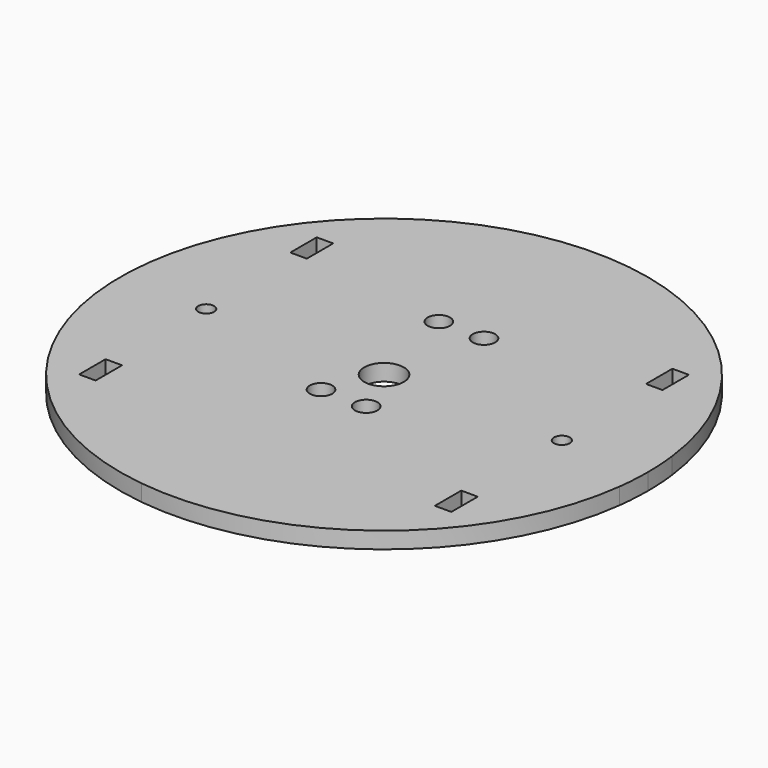
from build123d import *

# Parameters (mm, degrees)
F0_W     = 3.175
F0_H     = 6.35
F0_R     = 1.524
F0_R_2   = 2.159
F0_R_3   = 3.81
F1_DEPTH = 3.175


# Not quite as in the source:
# - a length typed as a fraction of an inch, garbled in the dataset ("3 / 203.2 mm" for 3/8 in), is restored


with BuildPart() as f1:
    # F0 (on Top) → F1 (new body)
    with BuildSketch(Plane.XY):
        with BuildLine():
            ThreePointArc((-50.403125, 6.3375855209), (-50.8, 0), (-50.403125, -6.3375855209))
            ThreePointArc((-50.403125, -6.3375855209), (-35.9210244843, -35.9210244843), (-6.3375855209, -50.403125))
            ThreePointArc((-6.3375855209, -50.403125), (0, -50.8), (6.3375855209, -50.403125))
            ThreePointArc((6.3375855209, -50.403125), (35.9210244843, -35.9210244843), (50.403125, -6.3375855209))
            ThreePointArc((50.403125, -6.3375855209), (50.700684167, -3.175), (50.8, 0))
            ThreePointArc((50.8, 0), (50.700684167, 3.175), (50.403125, 6.3375855209))
            ThreePointArc((50.403125, 6.3375855209), (35.9210244843, 35.9210244843), (6.3375855209, 50.403125))
            ThreePointArc((6.3375855209, 50.403125), (0, 50.8), (-6.3375855209, 50.403125))
            ThreePointArc((-6.3375855209, 50.403125), (-35.9210244843, 35.9210244843), (-50.403125, 6.3375855209))
        make_face()
        with Locations((-34.2304483056, -25.4)):
            Rectangle(F0_W, F0_H, mode=Mode.SUBTRACT)
        with Locations((-34.2304483056, 0)):
            Circle(F0_R, mode=Mode.SUBTRACT)
        with Locations((-4.3434, -9.7282)):
            Circle(F0_R_2, mode=Mode.SUBTRACT)
        Circle(F0_R_3, mode=Mode.SUBTRACT)
        with Locations((34.2304483056, -25.4)):
            Rectangle(F0_W, F0_H, mode=Mode.SUBTRACT)
        with Locations((4.3434, -9.7282)):
            Circle(F0_R_2, mode=Mode.SUBTRACT)
        with Locations((34.2304483056, 0)):
            Circle(F0_R, mode=Mode.SUBTRACT)
        with Locations((-34.2304483056, 25.4)):
            Rectangle(F0_W, F0_H, mode=Mode.SUBTRACT)
        with Locations((-4.3434, 18.6182)):
            Circle(F0_R_2, mode=Mode.SUBTRACT)
        with Locations((4.3434, 18.6182)):
            Circle(F0_R_2, mode=Mode.SUBTRACT)
        with Locations((34.2304483056, 25.4)):
            Rectangle(F0_W, F0_H, mode=Mode.SUBTRACT)
    extrude(amount=F1_DEPTH)


solid = f1.part
